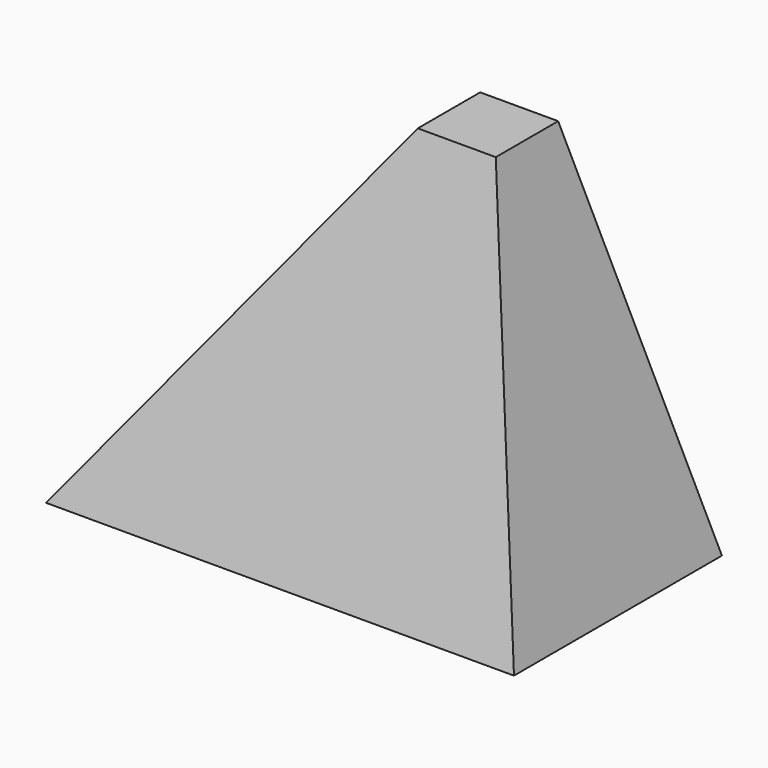
from build123d import *

# Parameters (mm, degrees)
F1_DEPTH = 25
F2_SIZE2 = 74.99999
F2_SIZE  = 17.49999


# Not quite as in the source:
# - a fillet or chamfer is up to 0.001 mm smaller than in the source, because OpenCascade refuses the exact size


with BuildPart() as f1:
    # F0 (on Front) → F1 (new body, symmetric)
    with BuildSketch(Plane.XZ):
        Polygon((25, -29.9881670944), (7.5, 45.0118329056), (-7.5, 45.0118329056), (-65, -29.9881670944), (-25, -29.9881670944), align=None)
    extrude(amount=F1_DEPTH, both=True)

    # F2 (size 17.5 and 75 in the source; OpenCascade refuses exactly that, so slightly less here)
    f2_edges = [f1.edges().sort_by_distance(p)[0] for p in [
        (0, 25, 45.011833),
        (0, -25, 45.011833),
    ]]
    f2_side = f1.faces().sort_by_distance((0, 0, 45.011833))[0]
    chamfer(f2_edges, length=F2_SIZE, length2=F2_SIZE2, reference=f2_side)


solid = f1.part
